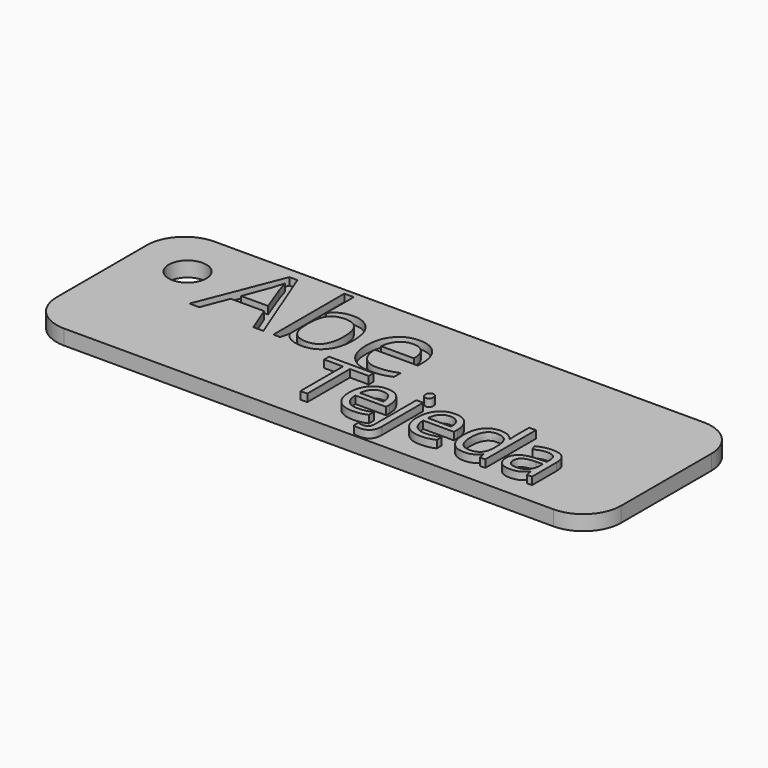
from build123d import *

# Parameters (mm, degrees)
F1_DEPTH     = 2
F3_D         = 5
F4_TEXT_SIZE = 15.5102836692
F5_DEPTH     = 1
F6_TEXT_SIZE = 11.0644530246
F7_DEPTH     = 1


# Not quite as in the source:
# - Text() gives the source's letters only with a copy of the font that has no kerning and outlines rounded to 1/6400 em; it was checked with that copy


with BuildPart() as f1:
    # F0 (on Top) → F1 (new body)
    with BuildSketch(Plane.XY):
        with BuildLine():
            Line((32.5, 12.5), (-32.5, 12.5))
            ThreePointArc((-32.5, 12.5), (-36.0355339059, 11.0355339059), (-37.5, 7.5))
            Line((-37.5, 7.5), (-37.5, -7.5))
            ThreePointArc((-37.5, -7.5), (-36.0355339059, -11.0355339059), (-32.5, -12.5))
            Line((-32.5, -12.5), (32.5, -12.5))
            ThreePointArc((32.5, -12.5), (36.0355339059, -11.0355339059), (37.5, -7.5))
            Line((37.5, -7.5), (37.5, 7.5))
            ThreePointArc((37.5, 7.5), (36.0355339059, 11.0355339059), (32.5, 12.5))
        make_face()
    extrude(amount=F1_DEPTH)

    # F3 (through all)
    with Locations(Plane.XY.offset(2)):
        with Locations((-30.5, 5.5)):
            Hole(F3_D / 2)

    # F4 (on face) → F5 (cut)
    with BuildSketch(Plane.XY.offset(2)):
        with Locations((-25.8467234671, 0)):
            Text('Abe', F4_TEXT_SIZE, font='Open Sans', text_align=(TextAlign.LEFT, TextAlign.BOTTOM))
    extrude(amount=-F5_DEPTH, mode=Mode.SUBTRACT)

    # F6 (on face) → F7 (join)
    with BuildSketch(Plane.XY.offset(2)):
        with Locations((-5.9820516035, -9.6616223454)):
            Text('Tejeda', F6_TEXT_SIZE, font='Open Sans', text_align=(TextAlign.LEFT, TextAlign.BOTTOM))
    extrude(amount=F7_DEPTH)


solid = f1.part
